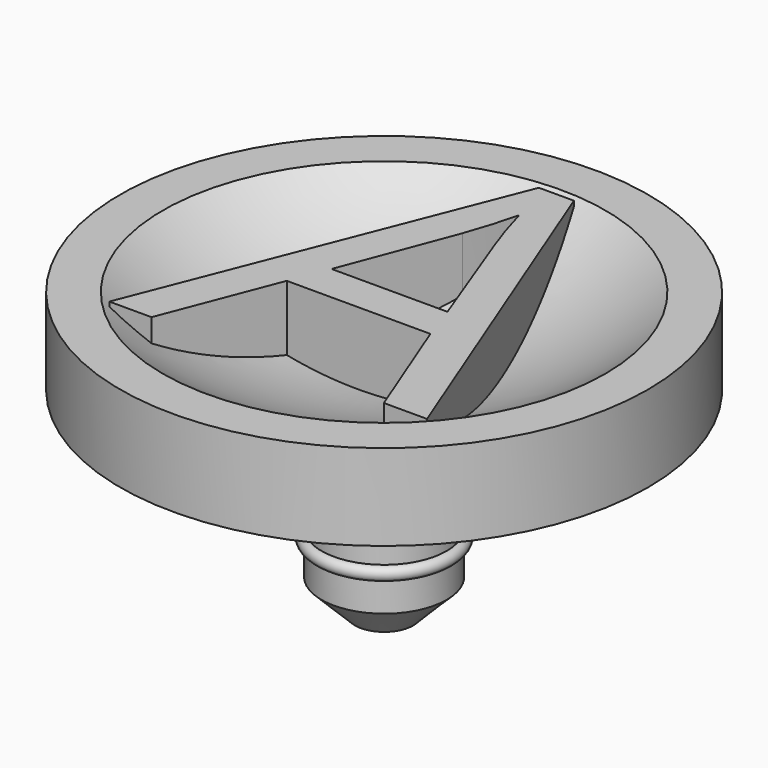
from build123d import *

# Parameters (mm, degrees)
F2_TEXT_SIZE = 19.0165314254
F3_DEPTH     = 4.064
F4_W         = 439.3387079644
F4_H         = 117.3384692084
F5_DEPTH     = 12.7
F6_SIZE      = 1.27
F7_R         = 18.576784554
F7_R_2       = 5.842
F8_DEPTH     = 0.8
F9_SIZE      = 1.016


# Not quite as in the source:
# - Text() gives the source's letters only with a copy of the font that has no kerning and outlines rounded to 1/6400 em; it was checked with that copy


with BuildPart() as f1:
    # F0 (on Front) → F1 (revolve)
    with BuildSketch(Plane.XZ):
        with BuildLine():
            Line((2.6757909362, 0), (4.2185683136, 0))
            Line((4.2185683136, 0), (10, 0))
            Line((10, 0), (10, 5.4849551513))
            ThreePointArc((10, 5.4849551513), (5.4259986852, 2.3667937844), (0, 1.27))
            Line((0, 1.27), (0, 0))
            Line((0, 0), (0, -6.7))
            Line((0, -6.7), (2.3710267587, -6.7))
            Line((2.3710267587, -6.7), (2.3710267587, -4.308))
            ThreePointArc((2.3710267587, -4.308), (2.6250267587, -4.054), (2.3710267587, -3.8))
            Line((2.3710267587, -3.8), (2.3710267587, 0))
            Line((2.3710267587, 0), (2.6757909362, 0))
        make_face()
    revolve(axis=Axis((0, 0, 0.635), (0, 0, -1)))

    # F2 (on Top) → F3 (join)
    with BuildSketch(Plane.XY):
        with Locations((-5.9659417602, -5.5547766387)):
            Text('A', F2_TEXT_SIZE, font='Open Sans', text_align=(TextAlign.LEFT, TextAlign.BOTTOM))
    extrude(amount=F3_DEPTH)

    # F4 (on Right) → F5 (cut, symmetric)
    with BuildSketch(Plane.YZ):
        with Locations((-1.8443567678, 62.7332346042)):
            Rectangle(F4_W, F4_H)
    extrude(amount=F5_DEPTH, both=True, mode=Mode.SUBTRACT)

    # F6
    f6_edges = [f1.edges().sort_by_distance(p)[0] for p in [
        (-2.371027, 0, -6.7),
    ]]
    chamfer(f6_edges, length=F6_SIZE)

    # F7 (on face) → F8 (cut)
    with BuildSketch(Plane(origin=(0, 0, 0), x_dir=(1, 0, 0), z_dir=(0, 0, -1))):
        Circle(F7_R)
        Circle(F7_R_2, mode=Mode.SUBTRACT)
    extrude(amount=-F8_DEPTH, mode=Mode.SUBTRACT)

    # F9
    f9_edges = [f1.edges().sort_by_distance(p)[0] for p in [
        (-2.371027, 0, 0),
    ]]
    chamfer(f9_edges, length=F9_SIZE)


solid = f1.part
